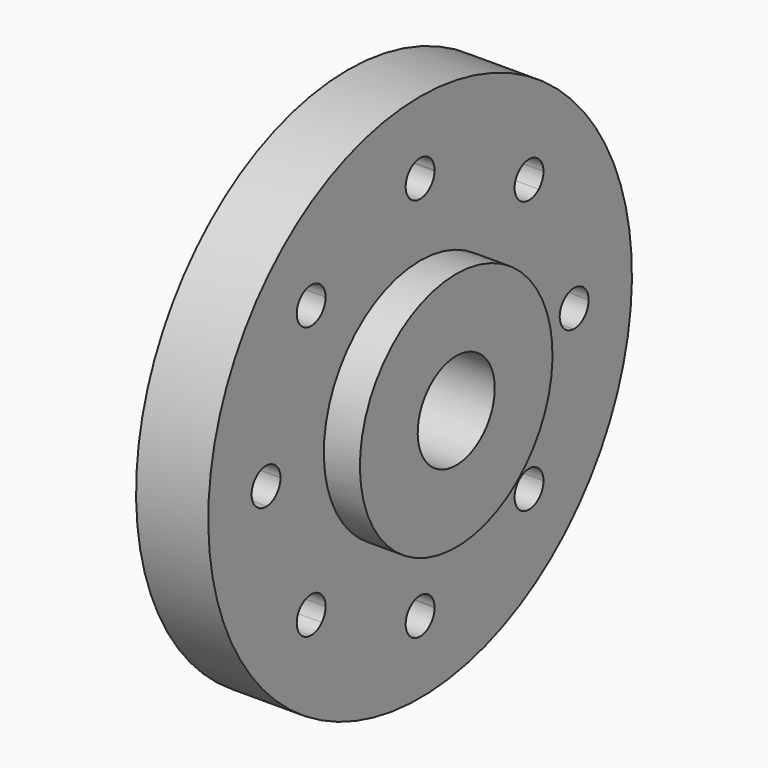
from build123d import *

# Parameters (mm, degrees)
F3_DEPTH = 50.801


with BuildPart() as f1:
    # F0 (on Front) → F1 (revolve)
    with BuildSketch(Plane.XZ):
        Polygon((0, 76.2), (0, 25.4), (69.85, 25.4), (69.85, 63.5), (50.8, 63.5), (50.8, 139.7), (12.7, 139.7), (12.7, 76.2), align=None)
    revolve(axis=Axis((-2.3766048754, 0, 0), (1, 0, 0)))

    # F2 (on face) → F3 (cut, through all)
    with BuildSketch(Plane.YZ.offset(50.8)):
        with BuildLine():
            ThreePointArc((9.5145297678, 101.153515625), (0, 101.6), (-9.5145297678, 101.153515625))
            ThreePointArc((-9.5145297678, 101.153515625), (0, 92.075), (9.5145297678, 101.153515625))
        make_face()
        with BuildLine():
            ThreePointArc((9.5145297678, 101.153515625), (9.5223820822, 101.3766964382), (9.525, 101.6))
            ThreePointArc((9.525, 101.6), (-0.2233035618, 111.1223820822), (-9.5145297678, 101.153515625))
            ThreePointArc((-9.5145297678, 101.153515625), (0, 101.6), (9.5145297678, 101.153515625))
        make_face()
        with BuildLine():
            ThreePointArc((-62.3170489686, 71.8420489686), (-62.9590604886, 75.2798012378), (-64.7985483207, 78.2541253579))
            ThreePointArc((-64.7985483207, 78.2541253579), (-71.8420489686, 71.8420489686), (-78.2541253579, 64.7985483207))
            ThreePointArc((-78.2541253579, 64.7985483207), (-67.9916855187, 63.1299696356), (-62.3170489686, 71.8420489686))
        make_face()
        with BuildLine():
            ThreePointArc((-78.2541253579, 64.7985483207), (-71.8420489686, 71.8420489686), (-64.7985483207, 78.2541253579))
            ThreePointArc((-64.7985483207, 78.2541253579), (-78.5772410594, 78.5772410594), (-78.2541253579, 64.7985483207))
        make_face()
        with BuildLine():
            ThreePointArc((-92.075, 0), (-94.7087595938, 6.5754414805), (-101.153515625, 9.5145297678))
            ThreePointArc((-101.153515625, 9.5145297678), (-101.6, 0), (-101.153515625, -9.5145297678))
            ThreePointArc((-101.153515625, -9.5145297678), (-94.7087595938, -6.5754414805), (-92.075, 0))
        make_face()
        with BuildLine():
            ThreePointArc((-101.153515625, -9.5145297678), (-101.6, 0), (-101.153515625, 9.5145297678))
            ThreePointArc((-101.153515625, 9.5145297678), (-111.125, 0), (-101.153515625, -9.5145297678))
        make_face()
        with BuildLine():
            ThreePointArc((-64.7985483207, -78.2541253579), (-71.8420489686, -71.8420489686), (-78.2541253579, -64.7985483207))
            ThreePointArc((-78.2541253579, -64.7985483207), (-78.5772410594, -78.5772410594), (-64.7985483207, -78.2541253579))
        make_face()
        with BuildLine():
            ThreePointArc((-62.3170489686, -71.8420489686), (-67.9916855187, -63.1299696356), (-78.2541253579, -64.7985483207))
            ThreePointArc((-78.2541253579, -64.7985483207), (-71.8420489686, -71.8420489686), (-64.7985483207, -78.2541253579))
            ThreePointArc((-64.7985483207, -78.2541253579), (-62.9590604886, -75.2798012378), (-62.3170489686, -71.8420489686))
        make_face()
        with BuildLine():
            ThreePointArc((9.5145297678, -101.153515625), (0, -92.075), (-9.5145297678, -101.153515625))
            ThreePointArc((-9.5145297678, -101.153515625), (0, -101.6), (9.5145297678, -101.153515625))
        make_face()
        with BuildLine():
            ThreePointArc((9.5145297678, -101.153515625), (0, -101.6), (-9.5145297678, -101.153515625))
            ThreePointArc((-9.5145297678, -101.153515625), (-0.2233035618, -111.1223820822), (9.525, -101.6))
            ThreePointArc((9.525, -101.6), (9.5223820822, -101.3766964382), (9.5145297678, -101.153515625))
        make_face()
        with BuildLine():
            ThreePointArc((81.3670489686, -71.8420489686), (80.5541283015, -67.9916855187), (78.2541253579, -64.7985483207))
            ThreePointArc((78.2541253579, -64.7985483207), (71.8420489686, -71.8420489686), (64.7985483207, -78.2541253579))
            ThreePointArc((64.7985483207, -78.2541253579), (75.2798012378, -80.7250374485), (81.3670489686, -71.8420489686))
        make_face()
        with BuildLine():
            ThreePointArc((64.7985483207, -78.2541253579), (71.8420489686, -71.8420489686), (78.2541253579, -64.7985483207))
            ThreePointArc((78.2541253579, -64.7985483207), (65.1068568778, -65.1068568778), (64.7985483207, -78.2541253579))
        make_face()
        with BuildLine():
            ThreePointArc((101.6, 0), (101.4883175235, 4.7625), (101.153515625, 9.5145297678))
            ThreePointArc((101.153515625, 9.5145297678), (92.075, 0), (101.153515625, -9.5145297678))
            ThreePointArc((101.153515625, -9.5145297678), (101.4883175235, -4.7625), (101.6, 0))
        make_face()
        with BuildLine():
            ThreePointArc((111.125, 0), (108.1754414805, 6.8912404062), (101.153515625, 9.5145297678))
            ThreePointArc((101.153515625, 9.5145297678), (101.4883175235, 4.7625), (101.6, 0))
            ThreePointArc((101.6, 0), (101.4883175235, -4.7625), (101.153515625, -9.5145297678))
            ThreePointArc((101.153515625, -9.5145297678), (108.1754414805, -6.8912404062), (111.125, 0))
        make_face()
        with BuildLine():
            ThreePointArc((81.3670489686, 71.8420489686), (75.2798012378, 80.7250374485), (64.7985483207, 78.2541253579))
            ThreePointArc((64.7985483207, 78.2541253579), (71.8420489686, 71.8420489686), (78.2541253579, 64.7985483207))
            ThreePointArc((78.2541253579, 64.7985483207), (80.5541283015, 67.9916855187), (81.3670489686, 71.8420489686))
        make_face()
        with BuildLine():
            ThreePointArc((78.2541253579, 64.7985483207), (71.8420489686, 71.8420489686), (64.7985483207, 78.2541253579))
            ThreePointArc((64.7985483207, 78.2541253579), (65.1068568778, 65.1068568778), (78.2541253579, 64.7985483207))
        make_face()
    extrude(amount=-F3_DEPTH, mode=Mode.SUBTRACT)


solid = f1.part
